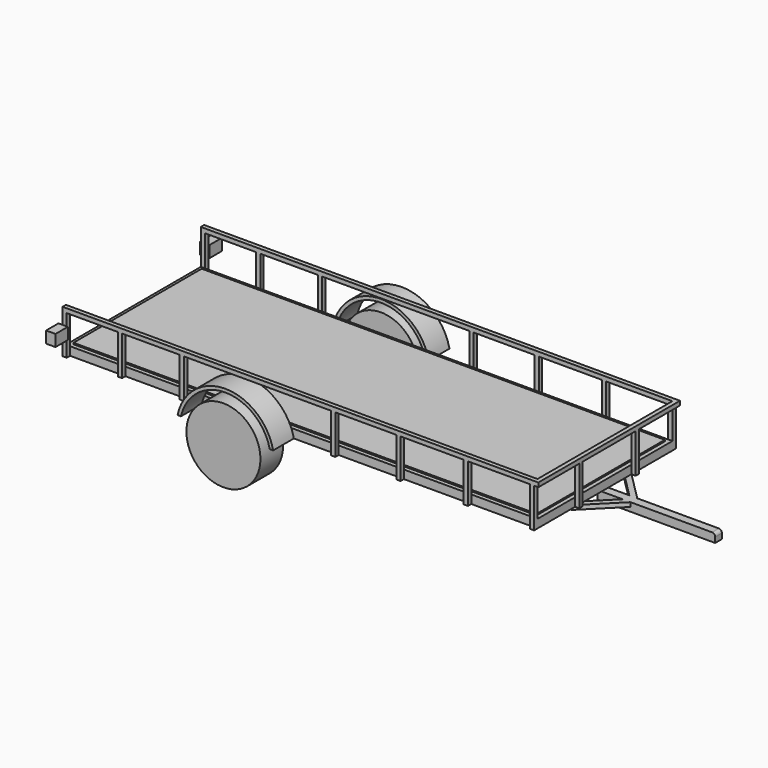
from build123d import *

# Parameters (mm, degrees)
F0_W      = 4266.9
F0_H      = 1526
F0_W_2    = 4190.7
F0_H_2    = 1449.8
F1_DEPTH  = 38.1
F2_DEPTH  = 50.8
F4_DEPTH  = 38.1
F6_DEPTH  = 38.1
F7_W      = 38.1
F7_H      = 38.1
F8_DEPTH  = 394
F10_DEPTH = 38.1
F11_W     = 85
F11_H     = 105
F12_DEPTH = 140
F13_R     = 335
F14_DEPTH = 256
F16_DEPTH = 234


# Not quite as in the source:
# - a pattern or mirror of a feature is missing from the dataset's text; its kind, count and spacing are read off the source's solid


with BuildPart() as f1:
    # F0 (on Top) → F1 (new body, symmetric)
    with BuildSketch(Plane.XY):
        Rectangle(F0_W, F0_H)
        Rectangle(F0_W_2, F0_H_2, mode=Mode.SUBTRACT)
    extrude(amount=F1_DEPTH, both=True)

    # F0 (on Top) → F2 (join)
    with BuildSketch(Plane.XY):
        Rectangle(F0_W_2, F0_H_2)
    extrude(amount=F2_DEPTH)

    # F3 (on Front) → F4 (join, symmetric)
    with BuildSketch(Plane.XZ):
        with BuildLine():
            Line((3133.45, -38.1), (2095.35, -38.1))
            Line((2095.35, -38.1), (2095.35, -114.3))
            Line((2095.35, -114.3), (3161.45, -114.3))
            Line((3161.45, -114.3), (3161.45, -66.1))
            ThreePointArc((3161.45, -66.1), (3153.2489898732, -46.3010101268), (3133.45, -38.1))
        make_face()
    extrude(amount=F4_DEPTH, both=True)

    # F5 (on face) → F6 (join)
    with BuildSketch(Plane.XY.offset(-38.1)):
        Polygon((2395.35, -38.1), (2323.5079510314, -38.1), (2095.35, -266.2579510314), (2095.35, -338.1), align=None)
    f6 = extrude(amount=-F6_DEPTH)

    # F6_copies: F6 across plane
    add(f6.mirror(Plane.ZX))

    # F7 (on face) → F8 (join)
    with BuildSketch(Plane(origin=(0, 0, -38.1), x_dir=(1, 0, 0), z_dir=(0, 0, -1))):
        with Locations((-2114.4, 782.05)):
            Rectangle(F7_W, F7_H)
        with Locations((-1614.4, 782.05)):
            Rectangle(F7_W, F7_H)
        with Locations((-1054.4, 782.05)):
            Rectangle(F7_W, F7_H)
        with Locations((315.6, 782.05)):
            Rectangle(F7_W, F7_H)
        with Locations((905.6, 782.05)):
            Rectangle(F7_W, F7_H)
        with Locations((1515.6, 782.05)):
            Rectangle(F7_W, F7_H)
        with Locations((2114.4, 782.05)):
            Rectangle(F7_W, F7_H)
        with Locations((2152.5, 319.05)):
            Rectangle(F7_W, F7_H)
    f8 = extrude(amount=-F8_DEPTH)

    # F8_copies: F8 across plane
    add(f8.mirror(Plane.ZX))

    # F9 (on face) → F10 (join)
    with BuildSketch(Plane.XY.offset(355.9)):
        Polygon((2133.45, 0), (2133.45, -763), (-2133.45, -763), (-2133.45, -801.1), (2171.55, -801.1), (2171.55, 0), align=None)
    f10 = extrude(amount=-F10_DEPTH)

    # F10_copies: F10 across plane
    add(f10.mirror(Plane.ZX))

    # F11 (on face) → F12 (join)
    with BuildSketch(Plane.XZ.offset(801.1)):
        with Locations((-2127.85, 159.4)):
            Rectangle(F11_W, F11_H)
    f12 = extrude(amount=F12_DEPTH)

    # F12_copies: F12 across plane
    add(f12.mirror(Plane.ZX))

    # F13 (on face) → F14 (join)
    with BuildSketch(Plane.XZ.offset(763)):
        with Locations((-503.45, -129.1)):
            Circle(F13_R)
    f14 = extrude(amount=F14_DEPTH)

    # F14_copies: F14 across plane
    add(f14.mirror(Plane.ZX))

    # F15 (on face) → F16 (join)
    with BuildSketch(Plane.XZ.offset(763)):
        with BuildLine():
            Line((-101.7279443446, -38.1), (-71.0212659871, -38.1))
            ThreePointArc((-71.0212659871, -38.1), (-503.45, 312.8), (-935.8787340129, -38.1))
            Line((-935.8787340129, -38.1), (-905.1720556554, -38.1))
            ThreePointArc((-905.1720556554, -38.1), (-503.45, 282.8), (-101.7279443446, -38.1))
        make_face()
    f16 = extrude(amount=F16_DEPTH)

    # F16_copies: F16 across plane
    add(f16.mirror(Plane.ZX))


solid = f1.part
